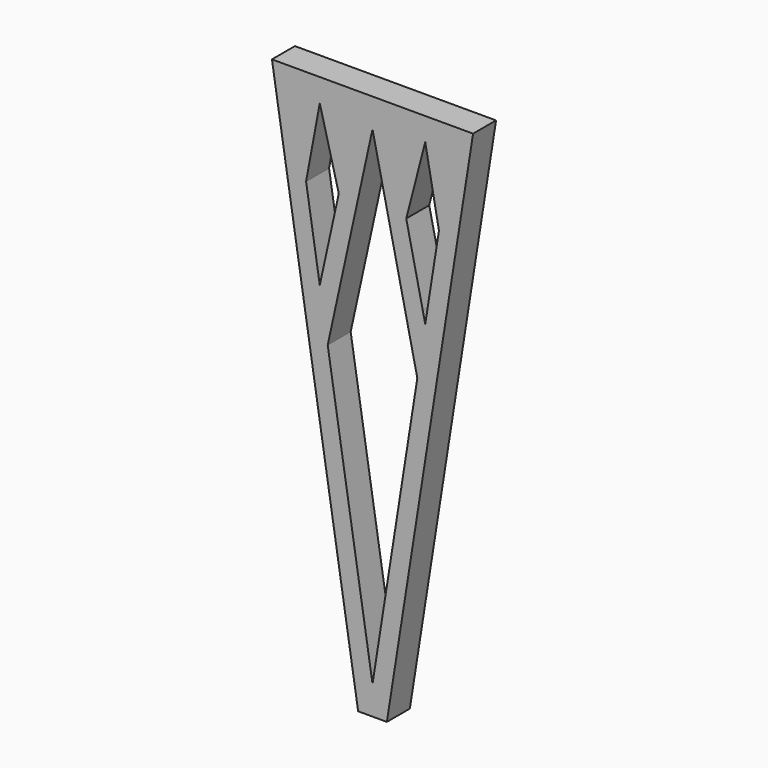
from build123d import *

# Parameters (mm, degrees)
F0_W      = 80
F0_H      = 16
F1_DEPTH  = 160
F3_DEPTH  = 25
F5_DEPTH  = 25
F7_W      = 70
F7_H      = 10
F8_DEPTH  = 190
F10_DEPTH = 25
F12_DEPTH = 25
F14_DEPTH = 25
F16_DEPTH = 25


with BuildPart() as f1:
    # F0 (on Top) → F1 (new body)
    with BuildSketch(Plane.XY):
        with Locations((40, 8)):
            Rectangle(F0_W, F0_H)
    extrude(amount=F1_DEPTH)

    # F2 (on face) → F3 (cut)
    with BuildSketch(Plane.XZ):
        Polygon((0, 160), (0, 0), (32.5, 0), align=None)
    extrude(amount=-F3_DEPTH, mode=Mode.SUBTRACT)

    # F4 (on face) → F5 (cut)
    with BuildSketch(Plane.XZ):
        Polygon((47.5, 0), (80, 0), (80, 160), align=None)
    extrude(amount=-F5_DEPTH, mode=Mode.SUBTRACT)


with BuildPart() as f8:
    # F7 (on Top) → F8 (new body)
    with BuildSketch(Plane.XY):
        with Locations((35, 5)):
            Rectangle(F7_W, F7_H)
    extrude(amount=F8_DEPTH)

    # F9 (on face) → F10 (cut)
    with BuildSketch(Plane.XZ):
        Polygon((0, 190), (0, 0), (30, 0), align=None)
    extrude(amount=-F10_DEPTH, mode=Mode.SUBTRACT)

    # F11 (on face) → F12 (cut)
    with BuildSketch(Plane.XZ):
        Polygon((40, 0), (70, 0), (70, 190), align=None)
    extrude(amount=-F12_DEPTH, mode=Mode.SUBTRACT)

    # F13 (on face) → F14 (cut)
    with BuildSketch(Plane.XZ):
        Polygon((19.4037426527, 108.7762965329), (35, 10), (50.5962573473, 108.7762965329), (35, 180), align=None)
    extrude(amount=-F14_DEPTH, mode=Mode.SUBTRACT)

    # F15 (on face) → F16 (cut)
    with BuildSketch(Plane.XZ):
        Polygon((11.8801091279, 156.4259755233), (16.6473853285, 126.2332262527), (17.4916778251, 130.0888716859), (23.2588624734, 156.4259755233), (16.6473853285, 181.9978654385), align=None)
        Polygon((58.1198908721, 156.4259755233), (53.3526146715, 181.9978654385), (46.7411375266, 156.4259755233), (52.5083221749, 130.0888716859), (53.3526146715, 126.2332262527), align=None)
    extrude(amount=-F16_DEPTH, mode=Mode.SUBTRACT)


solid = f8.part
